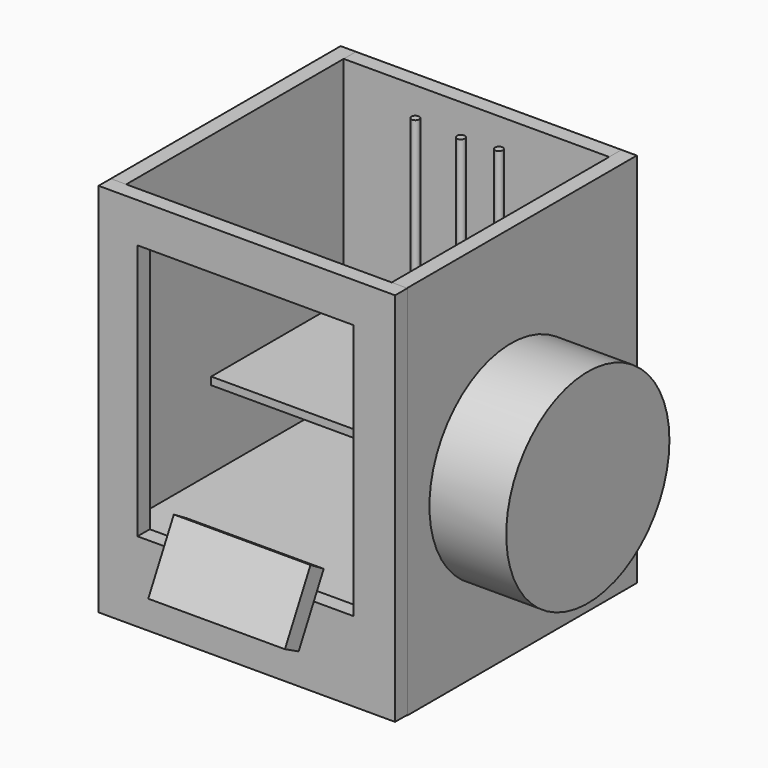
from build123d import *

# Parameters (mm, degrees)
F0_W      = 87.8305286169
F0_H      = 98.46470505
F1_DEPTH  = 5.08
F2_W      = 87.8305286169
F2_H      = 95.0086340308
F3_DEPTH  = 5.08
F4_W      = 95.0086340308
F4_H      = 124.5161257684
F5_DEPTH  = 5.08
F6_W      = 95.0086340308
F6_H      = 124.246340245
F7_DEPTH  = 5.08
F8_W      = 98.0914154202
F8_H      = 124.246340245
F9_DEPTH  = 5.08
F10_W     = 71.5218801051
F10_H     = 84.7484581172
F11_DEPTH = 25.4
F13_DEPTH = 11.43
F15_R     = 1.2840313407
F16_DEPTH = 92.964
F14_R     = 1.287825451
F17_DEPTH = 82.55
F18_W     = 37.7307755407
F18_H     = 56.4974024892
F19_DEPTH = 15.24
F20_W     = 21.343825385
F20_H     = 44.6666606003
F21_DEPTH = 9.144
F22_W     = 8.5665397346
F22_H     = 12.1454820037
F23_DEPTH = 25.4
F25_W     = 57.6052330434
F25_H     = 58.7303321809
F26_DEPTH = 2.54
F29_DEPTH = 45.212
F30_R     = 33.7449831522
F31_DEPTH = 25.4


with BuildPart() as f1:
    # F0 (on Front) → F1 (new body)
    with BuildSketch(Plane.XZ):
        with Locations((-6.466973573, 18.0510021746)):
            Rectangle(F0_W, F0_H)
    extrude(amount=F1_DEPTH)


with BuildPart() as f3:
    # F2 (on face) → F3 (new body)
    with BuildSketch(Plane(origin=(0, 0, -31.1813503504), x_dir=(1, 0, 0), z_dir=(0, 0, -1))):
        with Locations((-6.466973573, 47.5043170154)):
            Rectangle(F2_W, F2_H)
    extrude(amount=F3_DEPTH)

    # F22 (on face) → F23 (cut)
    with BuildSketch(Plane(origin=(0, 0, -36.2613503504), x_dir=(1, 0, 0), z_dir=(0, 0, -1))):
        with Locations((33.1650208682, 53.5770580173)):
            Rectangle(F22_W, F22_H)
    extrude(amount=-F23_DEPTH, mode=Mode.SUBTRACT)


with BuildPart() as f5:
    # F4 (on face) → F5 (new body)
    with BuildSketch(Plane.YZ.offset(37.4482907355)):
        with Locations((-47.5043170154, 5.0252918154)):
            Rectangle(F4_W, F4_H)
    extrude(amount=F5_DEPTH)


with BuildPart() as f7:
    # F6 (on face) → F7 (new body)
    with BuildSketch(Plane(origin=(-50.3822378814, 0, 0), x_dir=(0, -1, 0), z_dir=(-1, 0, 0))):
        with Locations((47.5043170154, 5.1601845771)):
            Rectangle(F6_W, F6_H)
    extrude(amount=F7_DEPTH)


with BuildPart() as f9:
    # F8 (on face) → F9 (new body)
    with BuildSketch(Plane.XZ.offset(95.0086340308)):
        with Locations((-6.4165301713, 5.1601845771)):
            Rectangle(F8_W, F8_H)
    extrude(amount=F9_DEPTH)

    # F10 (on face) → F11 (cut)
    with BuildSketch(Plane.XZ.offset(100.0886340308)):
        with Locations((-6.8259714171, 11.7521714419)):
            Rectangle(F10_W, F10_H)
    extrude(amount=-F11_DEPTH, mode=Mode.SUBTRACT)


with BuildPart() as f13:
    # F12 (on face) → F13 (new body)
    with BuildSketch(Plane.XZ.offset(5.08)):
        Polygon((-12.9339471459, -22.5257072598), (-6.466973573, -22.5257072598), (0, -22.5257072598), (0, -31.1813503504), (10.5579076335, -31.1813503504), (10.5579076335, -29.6559333801), (1.3164286502, -29.6559333801), (1.3164286502, -21.0573486984), (-6.466973573, -21.0573486984), (-14.2503757961, -21.0573486984), (-14.2503757961, -29.6559333801), (-23.4918547794, -29.6559333801), (-23.4918547794, -31.1813503504), (-12.9339471459, -31.1813503504), align=None)
    extrude(amount=F13_DEPTH)

    # F15 (on face) → F16 (join)
    with BuildSketch(Plane.XY.offset(-29.6559333801)):
        with Locations((-20.0384948403, -13.3861526847)):
            Circle(F15_R)
        with Locations((7.6200012118, -13.3861526847)):
            Circle(F15_R)
    extrude(amount=F16_DEPTH)


with BuildPart() as f17:
    # F14 (on face) → F17 (new body)
    with BuildSketch(Plane.XY.offset(-21.0573486984)):
        with Locations((-6.3092312776, -11.7070348933)):
            Circle(F14_R)
    extrude(amount=F17_DEPTH)


with BuildPart() as f19:
    # F18 (on face) → F19 (new body)
    with BuildSketch(Plane(origin=(0, 0, -36.2613503504), x_dir=(1, 0, 0), z_dir=(0, 0, -1))):
        with Locations((-29.2961454252, 63.908342272)):
            Rectangle(F18_W, F18_H)
    extrude(amount=F19_DEPTH)


with BuildPart() as f21:
    # F20 (on face) → F21 (new body)
    with BuildSketch(Plane(origin=(0, 0, -36.2613503504), x_dir=(1, 0, 0), z_dir=(0, 0, -1))):
        with Locations((24.4000153616, 24.1690996918)):
            Rectangle(F20_W, F20_H)
    extrude(amount=F21_DEPTH)


with BuildPart() as f26:
    # F25 (on offset) → F26 (new body)
    with BuildSketch(Plane.XY.offset(7.1726496496)):
        with Locations((-6.354464218, -49.529501237)):
            Rectangle(F25_W, F25_H)
    extrude(amount=F26_DEPTH)


with BuildPart() as f29:
    # F28 (on offset) → F29 (new body)
    with BuildSketch(Plane.YZ.offset(16.2131775388)):
        Polygon((-106.9532558322, -42.2394126654), (-96.5828751117, -22.3881331654), (-102.0563237106, -19.0516483007), (-112.6225219896, -39.277767374), align=None)
    extrude(amount=-F29_DEPTH)


with BuildPart() as f31:
    # F30 (on face) → F31 (new body)
    with BuildSketch(Plane.YZ.offset(42.5282907355)):
        with Locations((-52.0105399191, 0)):
            Circle(F30_R)
    extrude(amount=F31_DEPTH)


solid = Compound([f1.part, f3.part, f5.part, f7.part, f9.part, f13.part, f17.part, f19.part, f21.part, f26.part, f29.part, f31.part])
